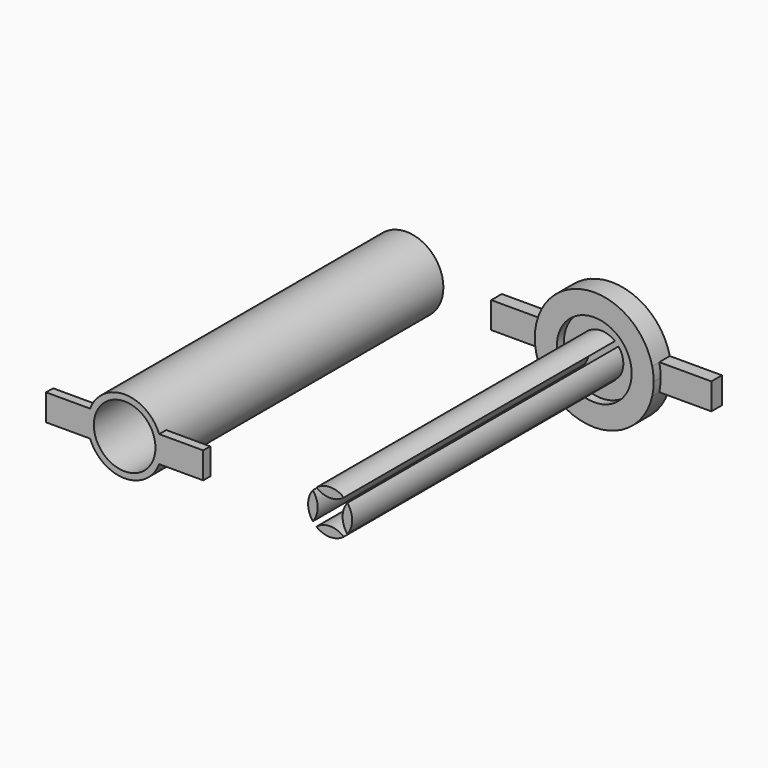
from build123d import *

# Parameters (mm, degrees)
F0_R      = 15.875
F1_DEPTH  = 3.81
F2_R      = 10.795
F3_DEPTH  = 2.54
F4_R      = 10.668
F4_R_2    = 8.89
F5_DEPTH  = 101.6
F8_DEPTH  = 2.54
F11_DEPTH = 97.79


# Not quite as in the source:
# - a feature names something its author has since deleted; it is built from what else it names


with BuildPart() as f1:
    # F0 (on Front) → F1 (new body)
    with BuildSketch(Plane.XZ):
        with BuildLine():
            Line((34.2841744423, 3.81), (34.2841744423, 0))
            Line((34.2841744423, 0), (34.2841744423, -3.81))
            Line((34.2841744423, -3.81), (49.3178672843, -3.81))
            ThreePointArc((49.3178672843, -3.81), (48.8891744423, 0), (49.3178672843, 3.81))
            Line((49.3178672843, 3.81), (34.2841744423, 3.81))
        make_face()
        with BuildLine():
            Line((97.7841744423, 3.81), (82.7504816003, 3.81))
            ThreePointArc((82.7504816003, 3.81), (83.0716641521, 1.9170209671), (83.1791744423, 0))
            ThreePointArc((83.1791744423, 0), (83.0716641521, -1.9170209671), (82.7504816003, -3.81))
            Line((82.7504816003, -3.81), (97.7841744423, -3.81))
            Line((97.7841744423, -3.81), (97.7841744423, 0))
            Line((97.7841744423, 0), (97.7841744423, 3.81))
        make_face()
        with BuildLine():
            ThreePointArc((82.7504816003, 3.81), (66.0341744423, 17.145), (49.3178672843, 3.81))
            ThreePointArc((49.3178672843, 3.81), (48.8891744423, 0), (49.3178672843, -3.81))
            ThreePointArc((49.3178672843, -3.81), (66.0341744423, -17.145), (82.7504816003, -3.81))
            ThreePointArc((82.7504816003, -3.81), (83.0716641521, -1.9170209671), (83.1791744423, 0))
            ThreePointArc((83.1791744423, 0), (83.0716641521, 1.9170209671), (82.7504816003, 3.81))
        make_face()
        with Locations((66.0341744423, 0)):
            Circle(F0_R, mode=Mode.SUBTRACT)
        with Locations((66.0341744423, 0)):
            Circle(F0_R)
    extrude(amount=F1_DEPTH)

    # F2 (on face) → F3 (join)
    with BuildSketch(Plane.XZ.offset(3.81)):
        with BuildLine():
            ThreePointArc((82.7504816003, 3.81), (66.0341744423, 17.145), (49.3178672843, 3.81))
            ThreePointArc((49.3178672843, 3.81), (48.8891744423, 0), (49.3178672843, -3.81))
            ThreePointArc((49.3178672843, -3.81), (66.0341744423, -17.145), (82.7504816003, -3.81))
            ThreePointArc((82.7504816003, -3.81), (83.0716641521, -1.9170209671), (83.1791744423, 0))
            ThreePointArc((83.1791744423, 0), (83.0716641521, 1.9170209671), (82.7504816003, 3.81))
        make_face()
        with Locations((66.0341744423, 0)):
            Circle(F2_R, mode=Mode.SUBTRACT)
    extrude(amount=F3_DEPTH)

    # F10 (on face) → F11 (join)
    with BuildSketch(Plane.XZ.offset(3.81)):
        with BuildLine():
            ThreePointArc((61.0627080612, -3.9127058819), (62.4412416802, 0.0378664845), (61.0627080612, 3.9884388509))
            ThreePointArc((61.0627080612, 3.9884388509), (59.6841744423, 0.0378664845), (61.0627080612, -3.9127058819))
        make_face()
        with BuildLine():
            ThreePointArc((62.0836020759, 5.0093328655), (66.0341744423, 3.6307992466), (69.9847468087, 5.0093328655))
            ThreePointArc((69.9847468087, 5.0093328655), (66.0341744423, 6.3878664845), (62.0836020759, 5.0093328655))
        make_face()
        with BuildLine():
            ThreePointArc((69.9847468087, -4.9335998966), (66.0341744423, -3.5550662776), (62.0836020759, -4.9335998966))
            ThreePointArc((62.0836020759, -4.9335998966), (66.0341744423, -6.3121335155), (69.9847468087, -4.9335998966))
        make_face()
        with BuildLine():
            ThreePointArc((71.0056408233, 3.9884388509), (69.6271072044, 0.0378664845), (71.0056408233, -3.9127058819))
            ThreePointArc((71.0056408233, -3.9127058819), (72.3841744423, 0.0378664845), (71.0056408233, 3.9884388509))
        make_face()
    extrude(amount=F11_DEPTH)


with BuildPart() as f5:
    # F4 (on Front) → F5 (new body)
    with BuildSketch(Plane.XZ):
        with Locations((6.7617367022, 0)):
            Circle(F4_R)
        with Locations((6.7617367022, 0)):
            Circle(F4_R_2, mode=Mode.SUBTRACT)
    extrude(amount=F5_DEPTH)

    # F7 (on face) → F8 (join)
    with BuildSketch(Plane.XZ.offset(101.6)):
        with BuildLine():
            ThreePointArc((-3.2027062828, -3.81), (-3.9062632978, 0), (-3.2027062828, 3.81))
            Line((-3.2027062828, 3.81), (-15.9027062828, 3.81))
            Line((-15.9027062828, 3.81), (-15.9027062828, -3.81))
            Line((-15.9027062828, -3.81), (-3.2027062828, -3.81))
        make_face()
        with BuildLine():
            Line((29.4261796871, 3.81), (16.7261796871, 3.81))
            ThreePointArc((16.7261796871, 3.81), (17.2523730452, 1.9372075569), (17.4297367022, 0))
            ThreePointArc((17.4297367022, 0), (17.2523730452, -1.9372075569), (16.7261796871, -3.81))
            Line((16.7261796871, -3.81), (29.4261796871, -3.81))
            Line((29.4261796871, -3.81), (29.4261796871, 3.81))
        make_face()
    extrude(amount=-F8_DEPTH)


solid = Compound([f1.part, f5.part])
